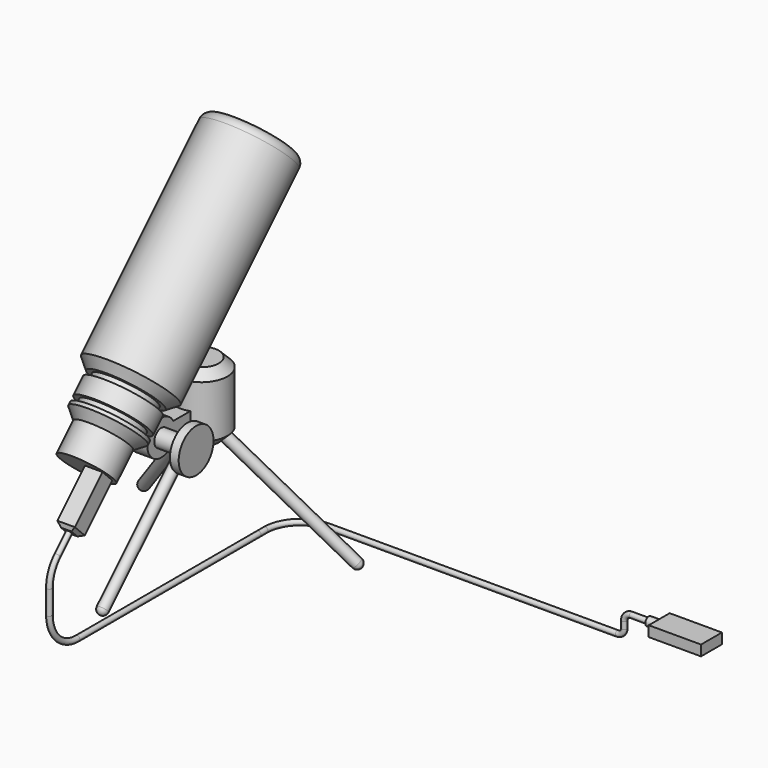
from build123d import *

# Parameters (mm, degrees)
F0_R      = 15
F1_DEPTH  = 40
F2_SIZE   = 5
F12_W     = 10
F12_H     = 10
F13_DEPTH = 30
F15_DEPTH = 5
F16_R     = 20
F17_DEPTH = 10
F20_R     = 5
F21_SIZE  = 4.99999
F22_R     = 5
F23_DEPTH = 15
F24_R     = 12.5
F25_DEPTH = 5
F26_W     = 10
F26_H     = 10
F27_DEPTH = 30
F28_SIZE  = 2
F30_R     = 1.5
F32_R     = 1.5
F36_R     = 1.5
F40_W     = 15
F40_H     = 6
F41_DEPTH = 30
F42_R     = 2.5
F43_DEPTH = 6


# Not quite as in the source:
# - a fillet or chamfer is up to 0.001 mm smaller than in the source, because OpenCascade refuses the exact size


with BuildPart() as f1:
    # F0 (on Top) → F1 (new body)
    with BuildSketch(Plane.XY):
        Circle(F0_R)
    extrude(amount=F1_DEPTH)

    # F2
    f2_edges = [f1.edges().sort_by_distance(p)[0] for p in [
        (-15, 0, 0),
        (-15, 0, 40),
    ]]
    chamfer(f2_edges, length=F2_SIZE)

    # F3 (on Right) → F4 (revolve)
    with BuildSketch(Plane.YZ):
        with BuildLine():
            Line((-2.1213203436, 14.1213203436), (-72.8319984622, -56.5893577751))
            ThreePointArc((-72.8319984622, -56.5893577751), (-73.7106781187, -58.7106781187), (-72.8319984622, -60.8319984622))
            Line((-72.8319984622, -60.8319984622), (0, 12))
            Line((0, 12), (-2.1213203436, 14.1213203436))
        make_face()
    revolve(axis=Axis((0, -36.4159992311, -24.4159992311), (0, 0.7071067812, 0.7071067812)))

    # F7 (on line) → F8 (revolve)
    with BuildSketch(Plane(origin=(0, 0, 0), x_dir=(0.8660254038, 0.5, 0), z_dir=(0.5, -0.8660254038, 0))):
        with BuildLine():
            Line((2.0230960578, 14.2195446293), (0, 12))
            Line((0, 12), (72.7337741765, -60.7337741765))
            ThreePointArc((72.7337741765, -60.7337741765), (73.6124538329, -58.6124538329), (72.7337741765, -56.4911334894))
            Line((72.7337741765, -56.4911334894), (2.0230960578, 14.2195446293))
        make_face()
    revolve(axis=Axis((31.494648075, 18.1834435441, -24.3668870882), (0.6123724357, 0.3535533906, -0.7071067812)))

    # F10 (on face) → F11 (revolve)
    with BuildSketch(Plane(origin=(0, 0, 0), x_dir=(0.8660254038, -0.5, 0), z_dir=(-0.5, -0.8660254038, 0))):
        with BuildLine():
            Line((-72.8869811403, -60.8869811403), (0, 12))
            Line((0, 12), (-2.1763030217, 14.0663376655))
            Line((-2.1763030217, 14.0663376655), (-72.8869811403, -56.6443404532))
            ThreePointArc((-72.8869811403, -56.6443404532), (-73.7656607968, -58.7656607968), (-72.8869811403, -60.8869811403))
        make_face()
    revolve(axis=Axis((-31.5609886363, 18.2217452851, -24.4434905702), (-0.6123724357, 0.3535533906, -0.7071067812)))

    # F12 (on Front) → F13 (join)
    with BuildSketch(Plane.XZ):
        with Locations((0, 15)):
            Rectangle(F12_W, F12_H)
    extrude(amount=F13_DEPTH)

    # F14 (on Right) → F15 (join, symmetric)
    with BuildSketch(Plane.YZ):
        with BuildLine():
            ThreePointArc((-44.6592582629, 17.588190451), (-36.3052619222, 5.0855513863), (-25, 15))
            ThreePointArc((-25, 15), (-28.9123857099, 22.9335334029), (-37.588190451, 24.6592582629))
            Line((-37.588190451, 24.6592582629), (-31.4644660941, 18.5355339059))
            Line((-31.4644660941, 18.5355339059), (-35, 15))
            Line((-35, 15), (-38.5355339059, 11.4644660941))
            Line((-38.5355339059, 11.4644660941), (-44.6592582629, 17.588190451))
        make_face()
        with BuildLine():
            Line((-31.4644660941, 18.5355339059), (-37.588190451, 24.6592582629))
            ThreePointArc((-37.588190451, 24.6592582629), (-42.0710678119, 22.0710678119), (-44.6592582629, 17.588190451))
            Line((-44.6592582629, 17.588190451), (-38.5355339059, 11.4644660941))
            Line((-38.5355339059, 11.4644660941), (-35, 15))
            Line((-35, 15), (-31.4644660941, 18.5355339059))
        make_face()
        with BuildLine():
            ThreePointArc((-44.6592582629, 17.588190451), (-42.0710678119, 22.0710678119), (-37.588190451, 24.6592582629))
            Line((-37.588190451, 24.6592582629), (-45.6066017178, 32.6776695297))
            Line((-45.6066017178, 32.6776695297), (-52.6776695297, 25.6066017178))
            Line((-52.6776695297, 25.6066017178), (-44.6592582629, 17.588190451))
        make_face()
    extrude(amount=F15_DEPTH, both=True)

    # F16 (on face) → F17 (join)
    with BuildSketch(Plane(origin=(0, -6.4644660941, -6.4644660941), x_dir=(1, 0, 0), z_dir=(0, 0.7071067812, 0.7071067812))):
        with Locations((0, -70.3553390593)):
            Circle(F16_R)
    extrude(amount=-F17_DEPTH)

    # F18 (on Right) → F19 (revolve)
    with BuildSketch(Plane.YZ):
        Polygon((-89.4472221514, 24.1923881554), (-82.3761543395, 17.1213203436), (37.8319984622, 137.3294731453), (20.1543289326, 155.0071426749), (-71.7695526217, 63.0832611207), (-66.1126983722, 57.4264068712), (-77.4264068712, 46.1126983722), (-79.5477272148, 48.2340187158), (-84.4974746831, 43.2842712475), (-80.9619407771, 39.7487373415), (-92.9827560573, 27.7279220614), align=None)
    revolve(axis=Axis((0, -22.2720779386, 77.2253967444), (0, 0.7071067812, 0.7071067812)))

    # F20
    f20_edges = [f1.edges().sort_by_distance(p)[0] for p in [
        (0, 55.509668, 119.651804),
    ]]
    fillet(f20_edges, radius=F20_R)

    # F21 (size 5 in the source; OpenCascade refuses exactly that, so slightly less here)
    f21_edges = [f1.edges().sort_by_distance(p)[0] for p in [
        (0, -36.414214, 27.727922),
        (0, -56.213203, 15),
    ]]
    chamfer(f21_edges, length=F21_SIZE)

    # F22 (on face) → F23 (join)
    with BuildSketch(Plane.YZ.offset(5)):
        with Locations((-35, 15)):
            Circle(F22_R)
    extrude(amount=F23_DEPTH)

    # F24 (on face) → F25 (join)
    with BuildSketch(Plane.YZ.offset(20)):
        with Locations((-35, 15)):
            Circle(F24_R)
    extrude(amount=F25_DEPTH)

    # F26 (on face) → F27 (join)
    with BuildSketch(Plane(origin=(0, -32.627416998, -32.627416998), x_dir=(1, 0, 0), z_dir=(0, -0.7071067812, -0.7071067812))):
        with Locations((7, 70.3553390593)):
            Rectangle(F26_W, F26_H)
    extrude(amount=F27_DEPTH)

    # F28
    f28_edges = [f1.edges().sort_by_distance(p)[0] for p in [
        (2, -103.589358, -4.091883),
        (7, -100.053824, -7.627417),
        (12, -103.589358, -4.091883),
        (7, -107.124892, -0.556349),
    ]]
    chamfer(f28_edges, length=F28_SIZE)

    # F31: sweep along a path in F29
    with BuildLine(Plane.YZ) as f31_path:
        Line((-103.5893577751, -4.091883092), (-111.8736290226, -12.3761543395))
        ThreePointArc((-111.8736290226, -12.3761543395), (-116.2090840491, -18.8646213159), (-117.7314933988, -26.5182899632))
        Line((-117.7314933988, -26.5182899632), (-117.7314933988, -40.2340187158))
        ThreePointArc((-117.7314933988, -40.2340187158), (-111.8736290226, -54.3761543395), (-97.7314933988, -60.2340187158))
        Line((-97.7314933988, -60.2340187158), (32.2685066012, -60.2340187158))
    # F30 (on face) → F31 (sweep)
    with BuildSketch(Plane(origin=(0, -53.8406204336, -53.8406204336), x_dir=(1, 0, 0), z_dir=(0, -0.7071067812, -0.7071067812))):
        with Locations((7, 70.3553390593)):
            Circle(F30_R)
    sweep(path=f31_path.line)

    # F35: sweep along a path in F34
    with BuildLine(Plane.XY.offset(-60.2340187158)) as f35_path:
        Line((177, 57.2685066012), (27, 57.2685066012))
        ThreePointArc((27, 57.2685066012), (12.8578643763, 51.4106422249), (7, 37.2685066012))
        Line((7, 37.2685066012), (7, 32.2685066012))
    # F32 (on face) → F35 (sweep)
    with BuildSketch(Plane(origin=(0, 32.2685066012, 0), x_dir=(-1, 0, 0), z_dir=(0, 1, 0))):
        with Locations((-7, -60.2340187158)):
            Circle(F32_R)
    sweep(path=f35_path.line)

    # F39: sweep along a path in F38
    with BuildLine(Plane(origin=(0, 57.2685066012, 0), x_dir=(-1, 0, 0), z_dir=(0, 1, 0))) as f39_path:
        Line((-177, -60.2340187158), (-193, -60.2340187158))
        ThreePointArc((-193, -60.2340187158), (-195.8284271247, -59.0624458405), (-197, -56.2340187158))
        Line((-197, -56.2340187158), (-197, -52.2340187158))
        ThreePointArc((-197, -52.2340187158), (-198.1715728753, -49.405591591), (-201, -48.2340187158))
        Line((-201, -48.2340187158), (-217, -48.2340187158))
    # F36 (on face) → F39 (sweep)
    with BuildSketch(Plane.YZ.offset(177)):
        with Locations((57.2685066012, -60.2340187158)):
            Circle(F36_R)
    sweep(path=f39_path.line)

    # F40 (on face) → F41 (join)
    with BuildSketch(Plane.YZ.offset(217)):
        with Locations((57.2685066012, -48.2340187158)):
            Rectangle(F40_W, F40_H)
    extrude(amount=F41_DEPTH)

    # F42 (on face) → F43 (join)
    with BuildSketch(Plane(origin=(217, 0, 0), x_dir=(0, -1, 0), z_dir=(-1, 0, 0))):
        with Locations((-57.2685066012, -48.2340187158)):
            Circle(F42_R)
    extrude(amount=F43_DEPTH)


solid = f1.part
